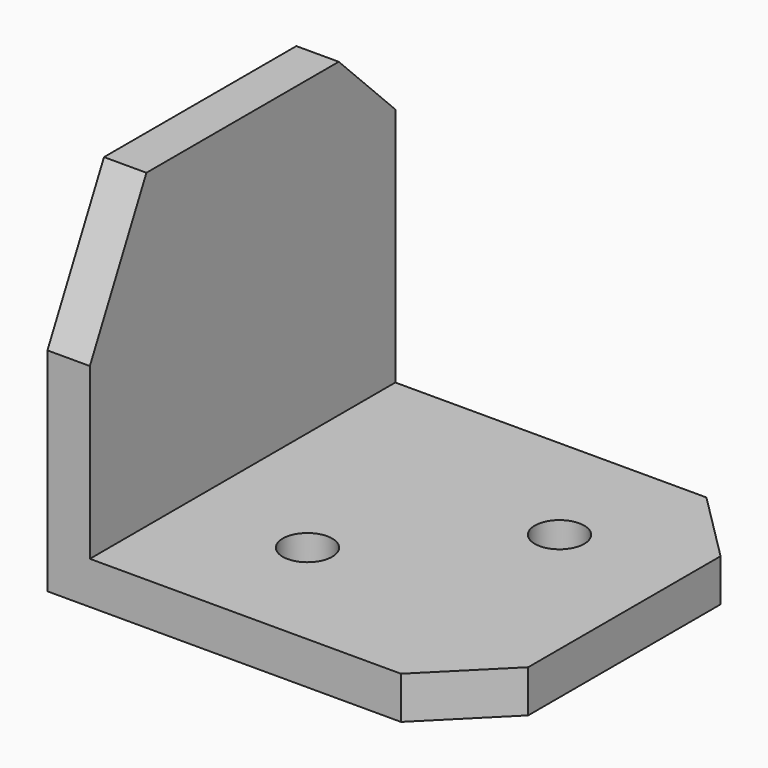
from build123d import *

# Parameters (mm, degrees)
F0_W     = 9.9
F0_H     = 4.9494949237
F1_DEPTH = 3
F0_W_2   = 3
F0_H_2   = 13.5
F2_DEPTH = 25
F3_D     = 3.5
F3_DEPTH = 12.4
F3_TIP   = 1.0515060833
F5_DEPTH = 30.001
F6_SIZE  = 5


# Not quite as in the source:
# - a feature names something its author has since deleted; it is built from what else it names


with BuildPart() as f1:
    # F0 (on Top) → F1 (new body)
    with BuildSketch(Plane.XY):
        with BuildLine():
            Line((25.4016518593, 6.6133860946), (-1.5983481407, 6.6133860946))
            Line((-1.5983481407, 6.6133860946), (-1.5983481407, -6.8866139054))
            Line((-1.5983481407, -6.8866139054), (4.9016518593, -6.8866139054))
            ThreePointArc((4.9016518593, -6.8866139054), (5.4344267975, -4.2079948582), (6.9516518593, -1.9371189817))
            ThreePointArc((6.9516518593, -1.9371189817), (11.9016518593, 0.1133860946), (16.8516518593, -1.9371189817))
            ThreePointArc((16.8516518593, -1.9371189817), (18.3688769211, -4.2079948582), (18.9016518593, -6.8866139054))
            Line((18.9016518593, -6.8866139054), (25.4016518593, -6.8866139054))
            Line((25.4016518593, -6.8866139054), (25.4016518593, 6.6133860946))
        make_face()
        with BuildLine():
            Line((4.9016518593, -6.8866139054), (-1.5983481407, -6.8866139054))
            Line((-1.5983481407, -6.8866139054), (-1.5983481407, -20.3866139054))
            Line((-1.5983481407, -20.3866139054), (25.4016518593, -20.3866139054))
            Line((25.4016518593, -20.3866139054), (25.4016518593, -6.8866139054))
            Line((25.4016518593, -6.8866139054), (18.9016518593, -6.8866139054))
            ThreePointArc((18.9016518593, -6.8866139054), (18.3688769211, -9.5652329526), (16.8516518593, -11.8361088292))
            ThreePointArc((16.8516518593, -11.8361088292), (11.9016518593, -13.8866139054), (6.9516518593, -11.8361088292))
            ThreePointArc((6.9516518593, -11.8361088292), (5.4344267975, -9.5652329526), (4.9016518593, -6.8866139054))
        make_face()
        with BuildLine():
            ThreePointArc((16.8516518593, -1.9371189817), (11.9016518593, 0.1133860946), (6.9516518593, -1.9371189817))
            Line((6.9516518593, -1.9371189817), (16.8516518593, -1.9371189817))
        make_face()
        with BuildLine():
            ThreePointArc((6.9516518593, -1.9371189817), (5.4344267975, -4.2079948582), (4.9016518593, -6.8866139054))
            Line((4.9016518593, -6.8866139054), (6.9516518593, -6.8866139054))
            Line((6.9516518593, -6.8866139054), (6.9516518593, -1.9371189817))
        make_face()
        with Locations((11.9016518593, -4.4118664436)):
            Rectangle(F0_W, F0_H)
        with BuildLine():
            Line((16.8516518593, -6.8866139054), (18.9016518593, -6.8866139054))
            ThreePointArc((18.9016518593, -6.8866139054), (18.3688769211, -4.2079948582), (16.8516518593, -1.9371189817))
            Line((16.8516518593, -1.9371189817), (16.8516518593, -6.8866139054))
        make_face()
        with BuildLine():
            ThreePointArc((16.8516518593, -11.8361088292), (18.3688769211, -9.5652329526), (18.9016518593, -6.8866139054))
            Line((18.9016518593, -6.8866139054), (16.8516518593, -6.8866139054))
            Line((16.8516518593, -6.8866139054), (16.8516518593, -11.8361088292))
        make_face()
        with Locations((11.9016518593, -9.3613613673)):
            Rectangle(F0_W, F0_H)
        with BuildLine():
            Line((6.9516518593, -6.8866139054), (4.9016518593, -6.8866139054))
            ThreePointArc((4.9016518593, -6.8866139054), (5.4344267975, -9.5652329526), (6.9516518593, -11.8361088292))
            Line((6.9516518593, -11.8361088292), (6.9516518593, -6.8866139054))
        make_face()
        with BuildLine():
            Line((16.8516518593, -11.8361088292), (6.9516518593, -11.8361088292))
            ThreePointArc((6.9516518593, -11.8361088292), (11.9016518593, -13.8866139054), (16.8516518593, -11.8361088292))
        make_face()
    extrude(amount=F1_DEPTH)

    # F0 (on Top) → F2 (join)
    with BuildSketch(Plane.XY):
        with Locations((-3.0983481407, -0.1366139054)):
            Rectangle(F0_W_2, F0_H_2)
        with Locations((-3.0983481407, -13.6366139054)):
            Rectangle(F0_W_2, F0_H_2)
    extrude(amount=F2_DEPTH)

    # F3
    with Locations(Plane(origin=(0, 0, 0), x_dir=(1, 0, 0), z_dir=(0, 0, -1))):
        with Locations((16.8516518593, 1.9371189817), (6.9516518593, 11.8361088292)):
            Hole(F3_D / 2, depth=F3_DEPTH)
            with Locations((0, 0, -(F3_DEPTH + F3_TIP / 2))):  # 118° drill point
                Cone(0, F3_D / 2, F3_TIP, mode=Mode.SUBTRACT)

    # F4 (on face) → F5 (cut, through all)
    with BuildSketch(Plane(origin=(-4.5983481407, 0, 0), x_dir=(0, -1, 0), z_dir=(-1, 0, 0))):
        Polygon((20.3866139054, 25), (15.3866139054, 25), (20.3866139054, 15), align=None)
    extrude(amount=-F5_DEPTH, mode=Mode.SUBTRACT)

    # F6
    f6_edges = [f1.edges().sort_by_distance(p)[0] for p in [
        (25.401652, -20.386614, 1.5),
        (25.401652, 6.613386, 1.5),
        (-3.098348, 6.613386, 25),
    ]]
    chamfer(f6_edges, length=F6_SIZE)


solid = f1.part
